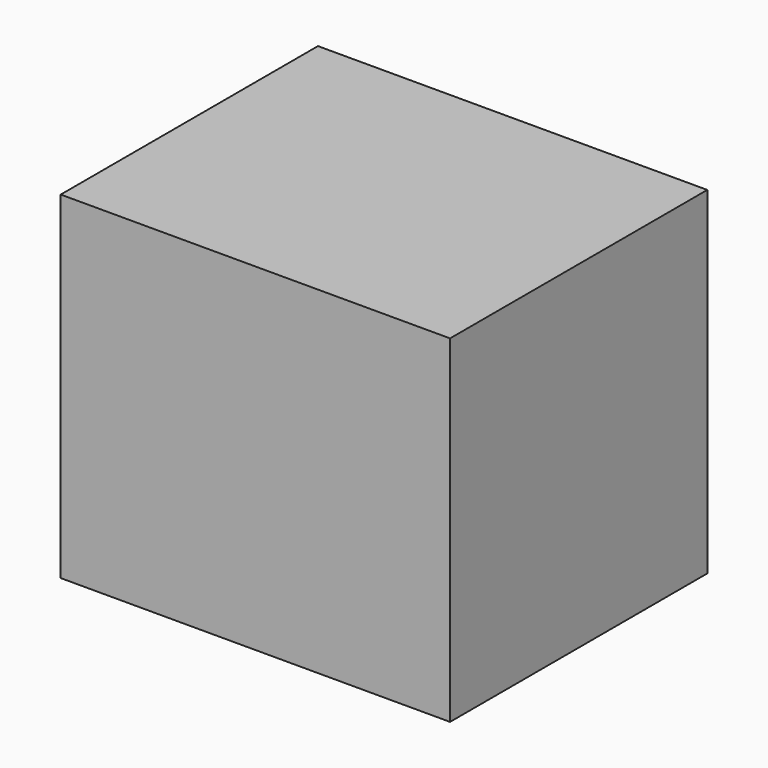
from build123d import *

# Parameters (mm, degrees)
F0_W          = 102.5072112679
F0_H          = 84.6536755562
F1_DEPTH      = 50.8
F1_DEPTH_BACK = 38.1


# Not quite as in the source:
# - the program builds the solid bodies; features that only make, move or delete a surface that nothing else refers to are left out


with BuildPart() as f1:
    # F0 (on Top) → F1 (new body, two sides)
    with BuildSketch(Plane.XY) as f1_sk:
        with Locations((51.253605634, -42.3268377781)):
            Rectangle(F0_W, F0_H)
    extrude(amount=F1_DEPTH)
    extrude(f1_sk.sketch, amount=-F1_DEPTH_BACK)


solid = f1.part
